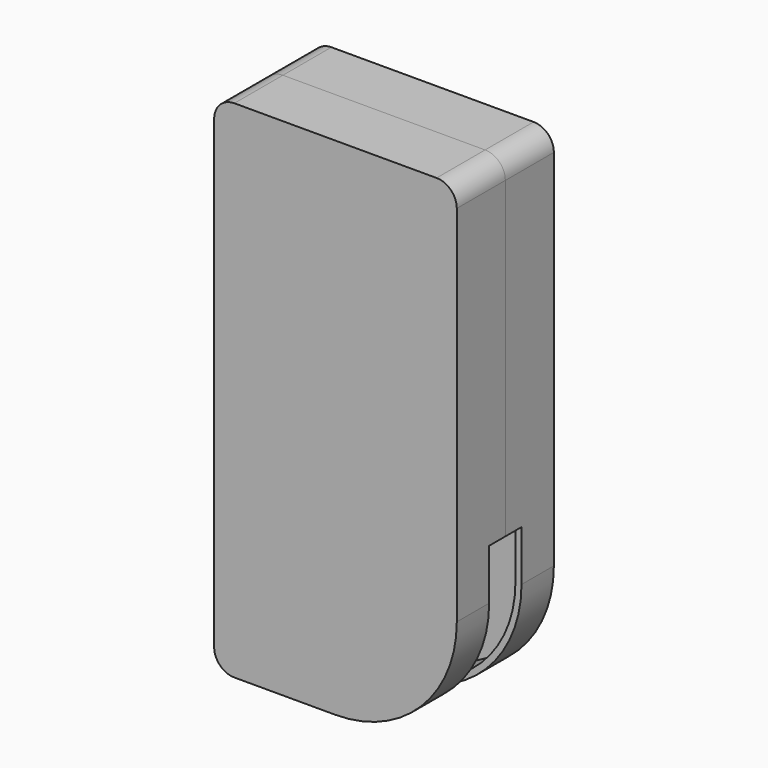
from build123d import *

# Parameters (mm, degrees)
F0_W      = 60
F0_H      = 125
F1_DEPTH  = 15
F2_R      = 5
F3_R      = 30
F4_T      = -1.5
F5_W      = 57
F5_H      = 1.5
F6_DEPTH  = 13.5
F7_R      = 9.5
F8_DEPTH  = 1.5
F9_W      = 1.5
F9_H      = 56
F10_DEPTH = 13.5
F11_R     = 2.5
F12_DEPTH = 13.5
F14_DEPTH = 1.5
F15_R     = 2.5
F16_DEPTH = 13.5
F18_DEPTH = 5


# Not quite as in the source:
# - a feature of the source that left no trace in its solid (it failed there, or was rolled back) is left out


with BuildPart() as f1:
    # F0 (on Front) → F1 (new body)
    with BuildSketch(Plane.XZ):
        with Locations((30, 62.5)):
            Rectangle(F0_W, F0_H)
    extrude(amount=F1_DEPTH)

    # F2
    f2_edges = [f1.edges().sort_by_distance(p)[0] for p in [
        (0, -7.5, 125),
        (60, -7.5, 125),
        (0, -7.5, 0),
    ]]
    fillet(f2_edges, radius=F2_R)

    # F3
    f3_edges = [f1.edges().sort_by_distance(p)[0] for p in [
        (60, -7.5, 0),
    ]]
    fillet(f3_edges, radius=F3_R)

    # F4
    f4_openings = [f1.faces().sort_by_distance(p)[0] for p in [
        (29.404035, -15, 63.933016),
    ]]
    offset(amount=F4_T, openings=f4_openings)

    # F5 (on face) → F6 (join, through all)
    with BuildSketch(Plane.XZ.offset(1.5)):
        with Locations((30, 66.75)):
            Rectangle(F5_W, F5_H)
    extrude(amount=F6_DEPTH)

    # F7 (on face) → F8 (cut, through all)
    with BuildSketch(Plane.XY.offset(67.5)):
        with Locations((23.5, -15)):
            Circle(F7_R)
    extrude(amount=-F8_DEPTH, mode=Mode.SUBTRACT)

    # F9 (on face) → F10 (join, through all)
    with BuildSketch(Plane.XZ.offset(1.5)):
        with Locations((37.75, 95.5)):
            Rectangle(F9_W, F9_H)
    extrude(amount=F10_DEPTH)

    # F11 (on face) → F12 (join, through all)
    with BuildSketch(Plane.XZ.offset(1.5)):
        with Locations((37.75, 66.75)):
            Circle(F11_R)
    extrude(amount=F12_DEPTH)

    # F13 (on face) → F14 (cut, through all)
    with BuildSketch(Plane(origin=(0, 0, 0), x_dir=(1, 0, 0), z_dir=(0, 0, -1))):
        with BuildLine():
            ThreePointArc((5, 15), (8, 12), (11, 15))
            Line((11, 15), (5, 15))
        make_face()
    extrude(amount=-F14_DEPTH, mode=Mode.SUBTRACT)

    # F15 (on face) → F16 (join, through all)
    with BuildSketch(Plane.XZ.offset(1.5)):
        with Locations((31, 27.5)):
            Circle(F15_R)
    extrude(amount=F16_DEPTH)

    # F17 (on face) → F18 (cut)
    with BuildSketch(Plane.XZ.offset(15)):
        with BuildLine():
            Line((60, 42.5), (31, 42.5))
            ThreePointArc((31, 42.5), (20.3933982822, 38.1066017178), (16, 27.5))
            Line((16, 27.5), (16, 0))
            Line((16, 0), (60, 0))
            Line((60, 0), (60, 42.5))
        make_face()
    extrude(amount=-F18_DEPTH, mode=Mode.SUBTRACT)


with BuildPart() as f19_1:
    # F19: instance of F1
    add(f1.part.mirror(Plane(origin=(28.1417704528, -15, 81.7211292347), x_dir=(1, 0, 0), z_dir=(0, -1, 0))))


solid = Compound([f1.part, f19_1.part])
